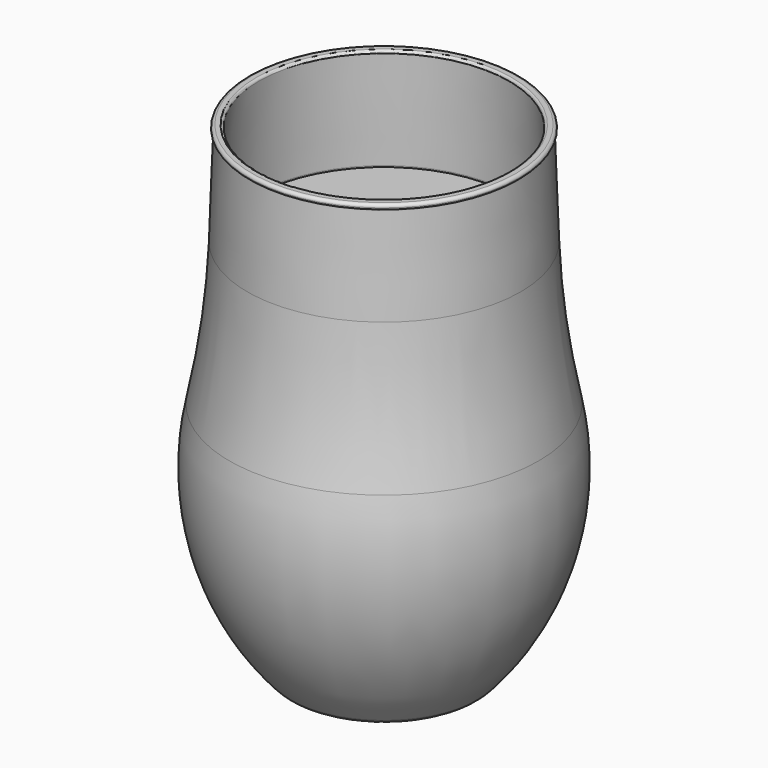
from build123d import *

# Parameters (mm, degrees)
F4_R      = 5
F5_R      = 3
F6_R      = 0.6
F9_R      = 3
F10_R     = 90.5961026067
F11_DEPTH = 26


with BuildPart() as f3:
    # F2 (on Front) → F3 (revolve)
    with BuildSketch(Plane.XZ):
        with BuildLine():
            Line((-31.1552316325, 59.99775), (-32.88138, 59.99775))
            ThreePointArc((-32.88138, 59.99775), (-33.4117100859, 59.7780800859), (-33.63138, 59.24775))
            ThreePointArc((-33.63138, 59.24775), (-33.4967324831, 58.8690059354), (-33.1532231118, 58.6602516969))
            ThreePointArc((-33.1532231118, 58.6602516969), (-33.1809688474, 58.5812577945), (-33.2086747351, 58.5022499072))
            Line((-33.2086747351, 58.5022499072), (-34.0495767416, 34.4219670651))
            ThreePointArc((-34.0495767416, 34.4219670651), (-35.4806511336, 16.5271388904), (-38.5105782621, -1.1672780515))
            ThreePointArc((-38.5105782621, -1.1672780515), (-37.5559106306, -32.6589214071), (-21.9041575982, -60.00225))
            Line((-21.9041575982, -60.00225), (-18, -60.00225))
            ThreePointArc((-18, -60.00225), (-9.1241437954, -57.7573872273), (0, -57.00225))
            Line((0, -57.00225), (0, -55.00225))
            ThreePointArc((0, -55.00225), (-9.2870878105, -55.7572061636), (-18.3303027798, -58.00225))
            Line((-18.3303027798, -58.00225), (-21.0434577329, -58.00225))
            ThreePointArc((-21.0434577329, -58.00225), (-35.7448305135, -31.7075056368), (-36.5564066232, -1.592969496))
            ThreePointArc((-36.5564066232, -1.592969496), (-33.4961802235, 16.2783916153), (-32.0507950875, 34.3521680717))
            Line((-32.0507950875, 34.3521680717), (-31.1552316325, 59.99775))
        make_face()
    revolve(axis=Axis((0, 0, -56.00225), (0, 0, 1)))

    # F4
    f4_edges = [f3.edges().sort_by_distance(p)[0] for p in [
        (21.904158, 0, -60.00225),
    ]]
    fillet(f4_edges, radius=F4_R)

    # F5
    f5_edges = [f3.edges().sort_by_distance(p)[0] for p in [
        (21.043458, 0, -58.00225),
    ]]
    fillet(f5_edges, radius=F5_R)

    # F6
    f6_edges = [f3.edges().sort_by_distance(p)[0] for p in [
        (31.155232, 0, 59.99775),
    ]]
    fillet(f6_edges, radius=F6_R)


with BuildPart() as f8:
    # F7 (on Front) → F8 (revolve)
    with BuildSketch(Plane.XZ):
        with BuildLine():
            ThreePointArc((-31.7765498208, 59.99775), (-31.3449459406, 59.8145450223), (-31.1769153246, 59.376810302))
            Line((-31.1769153246, 59.376810302), (-32.0507950875, 34.3521680717))
            ThreePointArc((-32.0507950875, 34.3521680717), (-33.4961802235, 16.2783916153), (-36.5564066232, -1.592969496))
            ThreePointArc((-36.5564066232, -1.592969496), (-35.7448305135, -31.7075056368), (-21.0434577329, -58.00225))
            Line((-21.0434577329, -58.00225), (-18.3303027798, -58.00225))
            ThreePointArc((-18.3303027798, -58.00225), (-9.2870878105, -55.7572061636), (0, -55.00225))
            Line((0, -55.00225), (0, 59.99775))
            Line((0, 59.99775), (-31.7765498208, 59.99775))
        make_face()
    revolve(axis=Axis((0, 0, 2.49775), (0, 0, 1)))

    # F9
    f9_edges = [f8.edges().sort_by_distance(p)[0] for p in [
        (21.043458, 0, -58.00225),
    ]]
    fillet(f9_edges, radius=F9_R)

    # F10 (on face) → F11 (cut)
    with BuildSketch(Plane.XY.offset(59.99775)):
        Circle(F10_R)
    extrude(amount=-F11_DEPTH, mode=Mode.SUBTRACT)


solid = Compound([f3.part, f8.part])
